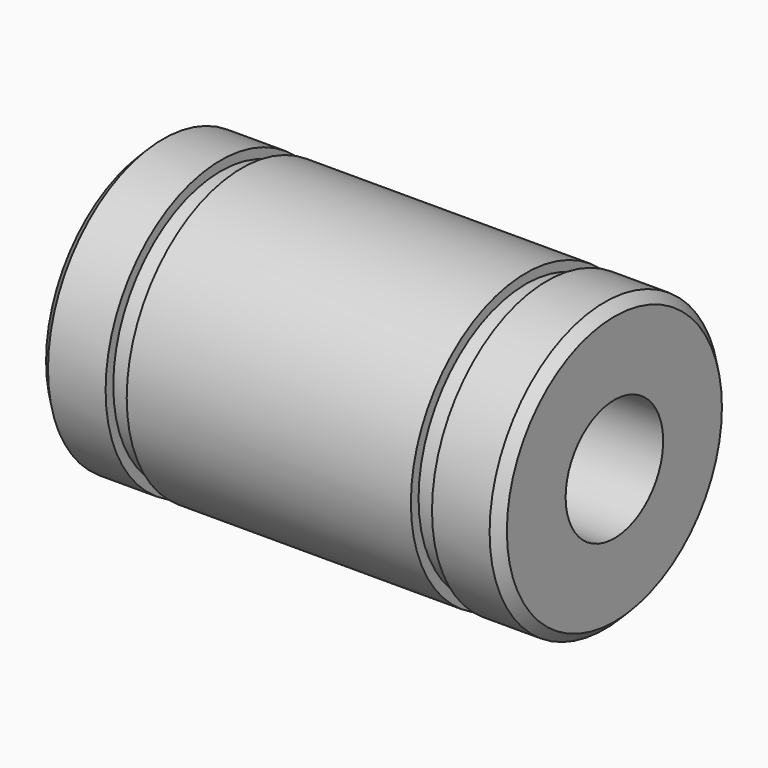
from build123d import *

# Parameters (mm, degrees)
F0_R     = 7.5
F1_DEPTH = 12
F3_D     = 6.35
F4_SIZE  = 0.5
F5_W     = 1.1
F5_H     = 3.9801998064


with BuildPart() as f1:
    # F0 (on Right) → F1 (new body, symmetric)
    with BuildSketch(Plane.YZ):
        Circle(F0_R)
    extrude(amount=F1_DEPTH, both=True)

    # F3 (through all)
    with Locations(Plane.YZ.offset(12)):
        with Locations((0, 0)):
            Hole(F3_D / 2)

    # F4
    f4_edges = [f1.edges().sort_by_distance(p)[0] for p in [
        (12, -7.5, 0),
        (-12, -7.5, 0),
        (-12, -3.175, 0),
    ]]
    chamfer(f4_edges, length=F4_SIZE)

    # F5 (on Front) → F6 (revolve, cut)
    with BuildSketch(Plane.XZ):
        with Locations((-7.95, 8.9900999032)):
            Rectangle(F5_W, F5_H)
        with Locations((7.95, 8.9900999032)):
            Rectangle(F5_W, F5_H)
    revolve(axis=Axis((-0.5466132425, 0, 0), (1, 0, 0)), mode=Mode.SUBTRACT)


solid = f1.part
